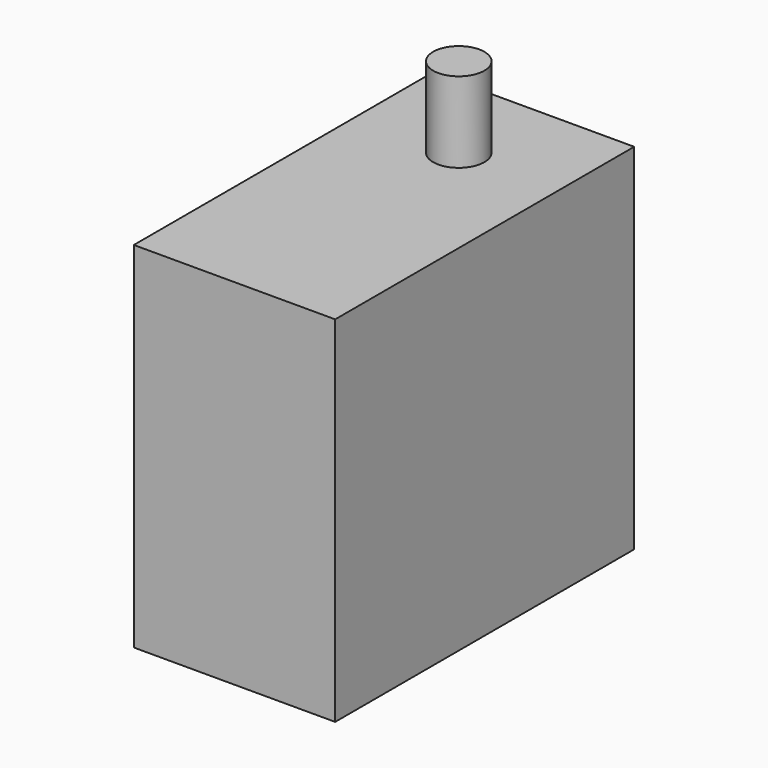
from build123d import *

# Parameters (mm, degrees)
F0_W     = 12.5
F0_H     = 23.2
F1_DEPTH = 22
F3_DEPTH = 5


with BuildPart() as f1:
    # F0 (on Top) → F1 (new body)
    with BuildSketch(Plane.XY):
        with Locations((-7.3471718132, 13.4849312573)):
            Rectangle(F0_W, F0_H)
    extrude(amount=F1_DEPTH)

    # F2 (on face) → F3 (join)
    with BuildSketch(Plane.XY.offset(22)):
        with BuildLine():
            ThreePointArc((-5.7571718132, 19.2849312573), (-7.3471718132, 20.8749312573), (-8.9371718132, 19.2849312573))
            Line((-8.9371718132, 19.2849312573), (-5.7571718132, 19.2849312573))
        make_face()
        with BuildLine():
            Line((-5.7571718132, 19.2849312573), (-8.9371718132, 19.2849312573))
            ThreePointArc((-8.9371718132, 19.2849312573), (-7.3471718132, 17.6949312573), (-5.7571718132, 19.2849312573))
        make_face()
    extrude(amount=F3_DEPTH)


solid = f1.part
